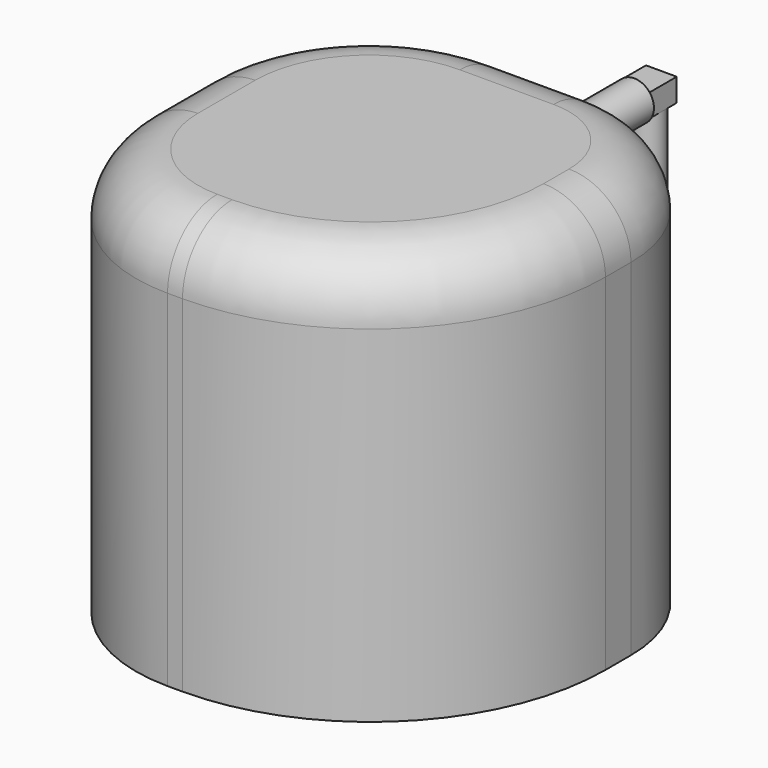
from build123d import *
from build123d import SkipClean  # not in build123d's __all__

# Parameters (mm, degrees)
F0_W         = 86.5733101964
F0_H         = 86.0464125872
F1_DEPTH     = 86.3111019135
F2_R         = 4.1730965083
F3_DEPTH     = 25.4
F5_DEPTH     = 7.1736387908
F6_R         = 3.3064136906
F7_DEPTH     = 43.7414944172
F9_DEPTH     = 8.9356992394
F10_R        = 2.3189722618
F11_DEPTH    = 25.4
F12_R        = 13.1155446623
F13_T1_DEPTH = 160.2242547154
F13_T4_ANGLE = 90
F14_T1_DEPTH = 179.2241870522
F14_T4_ANGLE = 90
F15_T1_DEPTH = 210.8662437018
F15_T4_ANGLE = 90
F16_T1_DEPTH = 170.7269310844
F16_T4_ANGLE = 90


# Not quite as in the source:
# - a fillet or chamfer that OpenCascade refuses, or shapes differently, is made with other operations: its cross-section is extruded or revolved along the edge and cut away or added


with BuildPart() as f1:
    # F0 (on Top) → F1 (new body)
    with BuildSketch(Plane.XY):
        with Locations((3.5064853728, -7.5555443764)):
            Rectangle(F0_W, F0_H)
    extrude(amount=F1_DEPTH)

    # F2 (on face) → F3 (join)
    with BuildSketch(Plane(origin=(0, 35.4676619172, 0), x_dir=(-1, 0, 0), z_dir=(0, 1, 0))):
        with Locations((-3.5064853728, 66.8797194958)):
            Circle(F2_R)
    extrude(amount=F3_DEPTH)

    # F4 (on face) → F5 (join)
    with BuildSketch(Plane(origin=(0, 60.8676619172, 0), x_dir=(-1, 0, 0), z_dir=(0, 1, 0))):
        with BuildLine():
            Line((-0.2548632519, 69.4953815632), (-6.7581074936, 69.4953815632))
            Line((-6.7581074936, 69.4953815632), (-6.7581074936, 64.6171336304))
            Line((-6.7581074936, 64.6171336304), (0, 64.6171336304))
            Line((0, 64.6171336304), (0, 69.1423053611))
            ThreePointArc((0, 69.1423053611), (-0.1228231667, 69.3221700158), (-0.2548632519, 69.4953815632))
        make_face()
    extrude(amount=F5_DEPTH)

    # F12
    f12_edges = [f1.edges().sort_by_distance(p)[0] for p in [
        (3.506485, 35.467662, 86.311102),
        (-39.78017, -7.555544, 86.311102),
        (3.506485, -50.578751, 86.311102),
        (46.79314, -7.555544, 86.311102),
    ]]
    fillet(f12_edges, radius=F12_R)

    # F13: fillet of radius 29.5652611208 on 1 edges, made by hand

    # F13_s2 → F13_t1 (cut)
    with BuildSketch(Plane.XY.offset(-73.9131528019)):
        with BuildLine():
            ThreePointArc((17.2278793502, 35.4676619172), (38.1336759763, 26.8081974225), (46.793140471, 5.9024007964))
            Line((46.793140471, 5.9024007964), (46.793140471, 35.4676619172))
            Line((46.793140471, 35.4676619172), (17.2278793502, 35.4676619172))
        make_face()
    extrude(amount=F13_T1_DEPTH, mode=Mode.SUBTRACT)

    # F13_s3 → F13_t4 (revolve, cut)
    with BuildSketch(Plane.XZ.offset(-5.9024007964)):
        with BuildLine():
            ThreePointArc((33.6775958086, 86.3111019135), (42.9516863783, 82.4696478208), (46.793140471, 73.1955572511))
            Line((46.793140471, 73.1955572511), (46.793140471, 86.3111019135))
            Line((46.793140471, 86.3111019135), (33.6775958086, 86.3111019135))
        make_face()
    revolve(axis=Axis((17.2278793502, 5.9024007964, 86.3111019135), (0, 0, 1)), revolution_arc=F13_T4_ANGLE, mode=Mode.SUBTRACT)

    # F14: fillet of radius 37.1652340555 on 1 edges, made by hand

    # F14_s2 → F14_t1 (cut)
    with BuildSketch(Plane.XY.offset(-92.9130851387)):
        with BuildLine():
            ThreePointArc((-2.6149356699, 35.4676619172), (-28.8947246949, 24.5822168867), (-39.7801697254, -1.6975721383))
            Line((-39.7801697254, -1.6975721383), (-39.7801697254, 35.4676619172))
            Line((-39.7801697254, 35.4676619172), (-2.6149356699, 35.4676619172))
        make_face()
    extrude(amount=F14_T1_DEPTH, mode=Mode.SUBTRACT)

    # F14_s3 → F14_t4 (revolve, cut)
    with BuildSketch(Plane.YZ.offset(-2.6149356699)):
        with BuildLine():
            ThreePointArc((22.3521172549, 86.3111019135), (31.6262078246, 82.4696478208), (35.4676619172, 73.1955572511))
            Line((35.4676619172, 73.1955572511), (35.4676619172, 86.3111019135))
            Line((35.4676619172, 86.3111019135), (22.3521172549, 86.3111019135))
        make_face()
    with SkipClean():  # cleaning this boolean's faces spoils the solid; the shape is the same uncleaned
        revolve(axis=Axis((-2.6149356699, -1.6975721383, 86.3111019135), (0, 0, 1)), revolution_arc=F14_T4_ANGLE, mode=Mode.SUBTRACT)

    # F15: fillet of radius 49.8221567152 on 1 edges, made by hand

    # F15_s2 → F15_t1 (cut)
    with BuildSketch(Plane.XY.offset(-124.5551417884)):
        with BuildLine():
            ThreePointArc((46.793240471, -0.7566939547), (32.2006686224, -35.9862788214), (-3.0289162443, -50.57885067))
            Line((-3.0289162443, -50.57885067), (-3.0289162443, -51.5752938043))
            ThreePointArc((-3.0289162443, -51.5752938043), (21.8821121134, -51.5751938043), (46.793140471, -51.5751938043))
            Line((46.793140471, -51.5751938043), (47.7895836053, -50.57875067))
            ThreePointArc((47.7895836053, -50.57875067), (47.7895836053, -25.6677223123), (47.7896836053, -0.7566939547))
            Line((47.7896836053, -0.7566939547), (46.793240471, -0.7566939547))
        make_face()
    extrude(amount=F15_T1_DEPTH, mode=Mode.SUBTRACT)

    # F15_s3 → F15_t4 (revolve, cut)
    with BuildSketch(Plane.YZ.offset(-3.0289162443)):
        with BuildLine():
            ThreePointArc((-37.4633060076, 86.3111019135), (-46.7373965773, 82.4696478208), (-50.57885067, 73.1955572511))
            Line((-50.57885067, 73.1955572511), (-50.57885067, 86.3111019135))
            Line((-50.57885067, 86.3111019135), (-37.4633060076, 86.3111019135))
        make_face()
    revolve(axis=Axis((-3.0289162443, -0.7566939547, 86.3111019135), (0, 0, 1)), revolution_arc=F15_T4_ANGLE, mode=Mode.SUBTRACT)

    # F16: fillet of radius 33.7664316682 on 1 edges, made by hand

    # F16_s2 → F16_t1 (cut)
    with BuildSketch(Plane.XY.offset(-84.415829171)):
        with BuildLine():
            ThreePointArc((-6.0138380572, -50.57885067), (-29.8903108663, -40.6888918108), (-39.7802697254, -16.8124190017))
            Line((-39.7802697254, -16.8124190017), (-40.4555983588, -16.8124190017))
            ThreePointArc((-40.4555983588, -16.8124190017), (-40.4554983588, -33.6955848358), (-40.4554983588, -50.57875067))
            Line((-40.4554983588, -50.57875067), (-39.7801697254, -51.2540793033))
            ThreePointArc((-39.7801697254, -51.2540793033), (-22.8970038913, -51.2540793033), (-6.0138380572, -51.2541793033))
            Line((-6.0138380572, -51.2541793033), (-6.0138380572, -50.57885067))
        make_face()
    extrude(amount=F16_T1_DEPTH, mode=Mode.SUBTRACT)

    # F16_s3 → F16_t4 (revolve, cut)
    with BuildSketch(Plane.XZ.offset(16.8124190017)):
        with BuildLine():
            ThreePointArc((-26.6647250631, 86.3111019135), (-35.9388156328, 82.4696478208), (-39.7802697254, 73.1955572511))
            Line((-39.7802697254, 73.1955572511), (-39.7802697254, 86.3111019135))
            Line((-39.7802697254, 86.3111019135), (-26.6647250631, 86.3111019135))
        make_face()
    revolve(axis=Axis((-6.0138380572, -16.8124190017, 86.3111019135), (0, 0, 1)), revolution_arc=F16_T4_ANGLE, mode=Mode.SUBTRACT)


with BuildPart() as f7:
    # F6 (on face) → F7 (new body)
    with BuildSketch(Plane(origin=(0, 0, 64.6171336304), x_dir=(1, 0, 0), z_dir=(0, 0, -1))):
        with Locations((3.4516938031, -64.4544813126)):
            Circle(F6_R)
    extrude(amount=F7_DEPTH)

    # F8 (on face) → F9 (join)
    with BuildSketch(Plane(origin=(0, 0, 20.8756392132), x_dir=(1, 0, 0), z_dir=(0, 0, -1))):
        with BuildLine():
            Line((0.7723765187, -62.5170525055), (0.7723765187, -66.3919101197))
            Line((0.7723765187, -66.3919101197), (6.0492576756, -66.3919101197))
            Line((6.0492576756, -66.3919101197), (6.0492576756, -62.4087458896))
            Line((6.0492576756, -62.4087458896), (0.8541299305, -62.4087458896))
            ThreePointArc((0.8541299305, -62.4087458896), (0.8126975418, -62.4624797498), (0.7723765187, -62.5170525055))
        make_face()
    extrude(amount=F9_DEPTH)

    # F10 (on face) → F11 (join)
    with BuildSketch(Plane.XZ.offset(-62.4087458896)):
        with Locations((3.6983042955, 15.4196098447)):
            Circle(F10_R)
    extrude(amount=F11_DEPTH)


solid = Compound([f1.part, f7.part])
